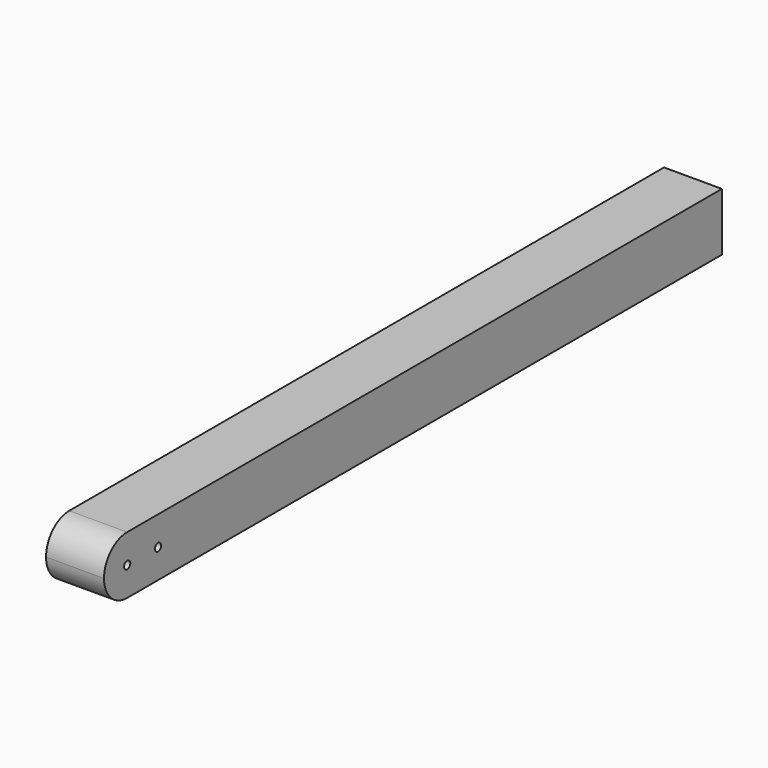
from build123d import *

# Parameters (mm, degrees)
F0_W     = 38.1
F0_H     = 38.1
F1_DEPTH = 508
F2_R     = 19.04999
F4_D     = 5.1054


# Not quite as in the source:
# - a fillet or chamfer is up to 0.001 mm smaller than in the source, because OpenCascade refuses the exact size


with BuildPart() as f1:
    # F0 (on Front) → F1 (new body)
    with BuildSketch(Plane.XZ):
        with Locations((-19.05, 19.05)):
            Rectangle(F0_W, F0_H)
    extrude(amount=F1_DEPTH)

    # F2 (radius 19.05 in the source; OpenCascade refuses exactly that, so slightly less here)
    f2_edges = [f1.edges().sort_by_distance(p)[0] for p in [
        (-19.05, -508, 38.1),
        (-19.05, -508, 0),
    ]]
    fillet(f2_edges, radius=F2_R)

    # F4 (through all)
    with Locations(Plane(origin=(-38.1, 0, 0), x_dir=(0, -1, 0), z_dir=(-1, 0, 0))):
        with Locations((488.95, 19.05), (463.55, 19.05)):
            Hole(F4_D / 2)


solid = f1.part
